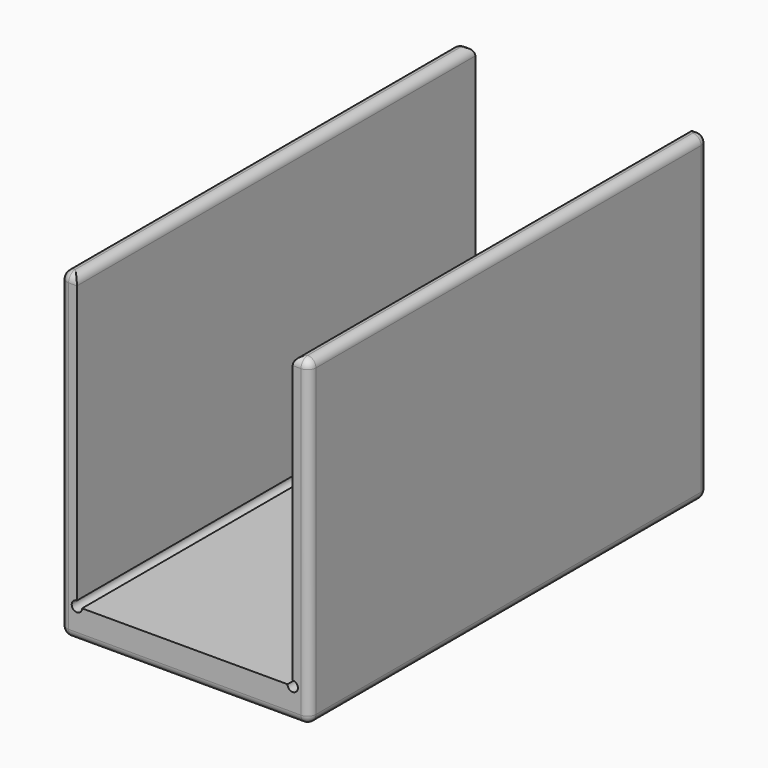
from build123d import *

# Parameters (mm, degrees)
F1_DEPTH = 76.2
F2_R     = 1.26999


# Not quite as in the source:
# - a fillet or chamfer is up to 0.001 mm smaller than in the source, because OpenCascade refuses the exact size


with BuildPart() as f1:
    # F0 (on Front) → F1 (new body)
    with BuildSketch(Plane.XZ):
        with BuildLine():
            Line((-16.51, 19.05), (-19.05, 19.05))
            Line((-19.05, 19.05), (-19.05, -30.1625))
            Line((-19.05, -30.1625), (0, -30.1625))
            Line((0, -30.1625), (0, -25.4))
            Line((0, -25.4), (-15.71625, -25.4))
            ThreePointArc((-15.71625, -25.4), (-17.0712660076, -25.9612660076), (-16.51, -24.60625))
            Line((-16.51, -24.60625), (-16.51, 19.05))
        make_face()
        with BuildLine():
            Line((0, -25.4), (0, -30.1625))
            Line((0, -30.1625), (19.05, -30.1625))
            Line((19.05, -30.1625), (19.05, 19.05))
            Line((19.05, 19.05), (16.51, 19.05))
            Line((16.51, 19.05), (16.51, -24.60625))
            ThreePointArc((16.51, -24.60625), (17.0712660076, -24.8387339924), (17.30375, -25.4))
            ThreePointArc((17.30375, -25.4), (16.51, -26.19375), (15.71625, -25.4))
            Line((15.71625, -25.4), (0, -25.4))
        make_face()
    extrude(amount=F1_DEPTH)

    # F2 (radius 1.27 in the source; OpenCascade refuses exactly that, so slightly less here)
    f2_edges = [f1.edges().sort_by_distance(p)[0] for p in [
        (19.05, -38.1, 19.05),
        (16.51, -38.1, 19.05),
        (17.78, 0, 19.05),
        (17.78, -76.2, 19.05),
        (-16.51, -38.1, 19.05),
        (-19.05, -38.1, 19.05),
        (-17.78, 0, 19.05),
        (-17.78, -76.2, 19.05),
        (-19.05, -76.2, -5.55625),
        (19.05, -76.2, -5.55625),
        (19.05, 0, -5.55625),
        (-19.05, 0, -5.55625),
        (-19.05, -38.1, -30.1625),
        (19.05, -38.1, -30.1625),
        (0, 0, -30.1625),
        (0, -76.2, -30.1625),
    ]]
    fillet(f2_edges, radius=F2_R)


solid = f1.part
